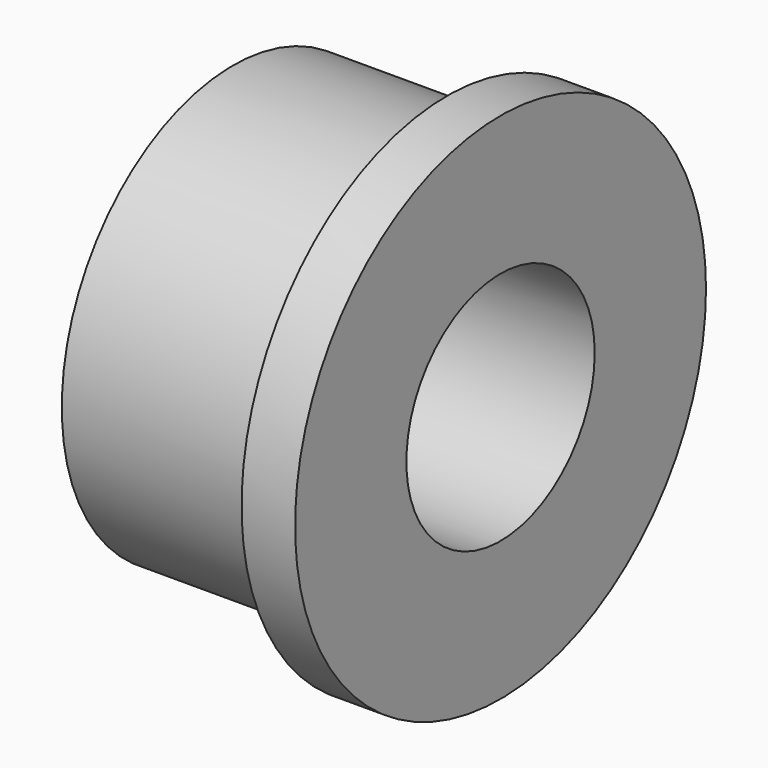
from build123d import *

# Parameters (mm, degrees)
F0_R     = 20
F0_R_2   = 11
F1_DEPTH = 25
F0_R_3   = 24
F2_DEPTH = 5


with BuildPart() as f1:
    # F0 (on Right) → F1 (new body)
    with BuildSketch(Plane.YZ):
        Circle(F0_R)
        Circle(F0_R_2, mode=Mode.SUBTRACT)
    extrude(amount=-F1_DEPTH)

    # F0 (on Right) → F2 (join)
    with BuildSketch(Plane.YZ):
        Circle(F0_R_3)
        Circle(F0_R, mode=Mode.SUBTRACT)
    extrude(amount=-F2_DEPTH)


solid = f1.part
